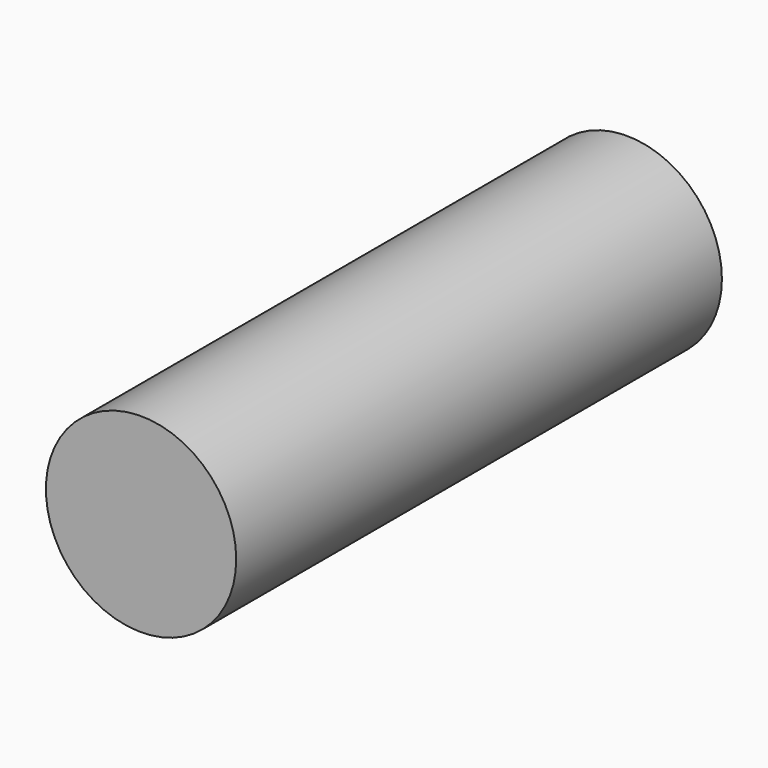
from build123d import *

# Parameters (mm, degrees)
F0_R     = 7.8365863053
F1_DEPTH = 50


# Not quite as in the source:
# - the program builds the solid bodies; features that only make, move or delete a surface that nothing else refers to are left out


with BuildPart() as f1:
    # F0 (on Front) → F1 (new body)
    with BuildSketch(Plane.XZ):
        with Locations((-55.8959804475, 48.7368889153)):
            Circle(F0_R)
    extrude(amount=F1_DEPTH)


solid = f1.part
